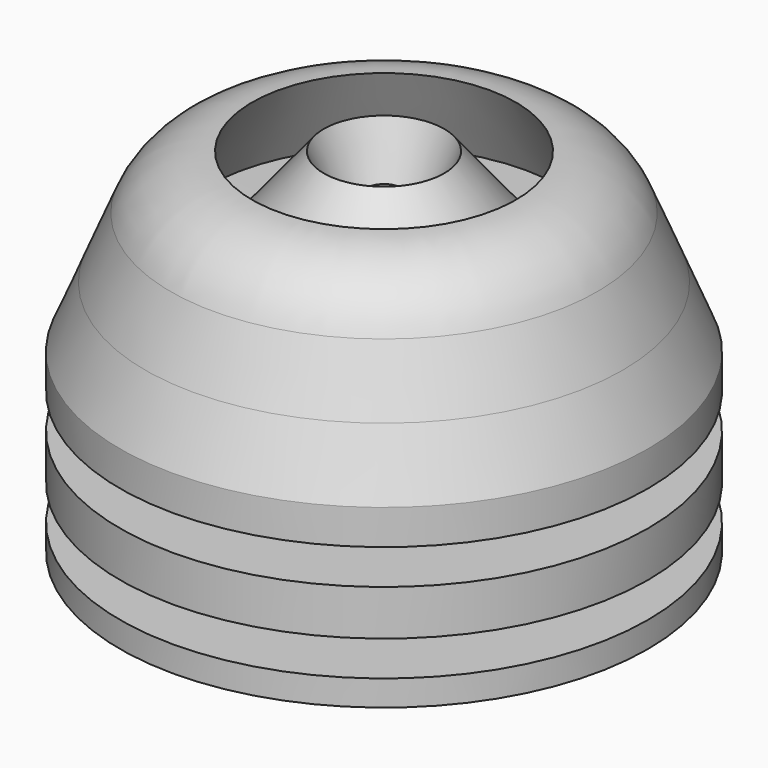
from build123d import *

# Parameters (mm, degrees)
F0_W   = 7.935712114
F0_H   = 3.1514726579
F0_W_2 = 16.216346994
F0_H_2 = 4.3113194406
F0_W_3 = 8.2806348801
F0_H_3 = 5.5851191282
F0_H_4 = 4.3113231659
F0_H_5 = 4.2968690395


with BuildPart() as f1:
    # F0 (on Right) → F1 (revolve)
    with BuildSketch(Plane.YZ):
        with Locations((20.184203051, 1.575736329)):
            Rectangle(F0_W, F0_H)
        with Locations((8.108173497, 5.3071323782)):
            Rectangle(F0_W_2, F0_H_2)
        with Locations((28.2923765481, 1.575736329)):
            Rectangle(F0_W_3, F0_H)
        with Locations((20.184203051, 5.3071323782)):
            Rectangle(F0_W, F0_H_2)
        with Locations((8.108173497, 10.2553516626)):
            Rectangle(F0_W_2, F0_H_3)
        with Locations((20.184203051, 10.2553516626)):
            Rectangle(F0_W, F0_H_3)
        with Locations((8.108173497, 15.2035728097)):
            Rectangle(F0_W_2, F0_H_4)
        with Locations((28.2923765481, 10.2553516626)):
            Rectangle(F0_W_3, F0_H_3)
        with Locations((20.184203051, 15.2035728097)):
            Rectangle(F0_W, F0_H_4)
        with Locations((8.108173497, 19.5076689124)):
            Rectangle(F0_W_2, F0_H_5)
        with Locations((20.184203051, 19.5076689124)):
            Rectangle(F0_W, F0_H_5)
        with BuildLine():
            Line((0, 39.0138179064), (0, 21.6561034322))
            Line((0, 21.6561034322), (16.216346994, 21.6561034322))
            Line((16.216346994, 21.6561034322), (16.216346994, 32.4841551483))
            Line((16.216346994, 32.4841551483), (7.3967017233, 43.3122068644))
            Line((7.3967017233, 43.3122068644), (3.9672423154, 34.0166091919))
            ThreePointArc((3.9672423154, 34.0166091919), (3.3885401848, 37.6305670459), (0, 39.0138179064))
        make_face()
        with Locations((28.2923765481, 19.5076689124)):
            Rectangle(F0_W_3, F0_H_5)
        with BuildLine():
            ThreePointArc((26.2175577062, 36.6341537335), (25.2214317596, 26.471239688), (16.216346994, 21.6561034322))
            Line((16.216346994, 21.6561034322), (24.152059108, 21.6561034322))
            Line((24.152059108, 21.6561034322), (32.4326939881, 21.6561034322))
            Line((32.4326939881, 21.6561034322), (29.3251258471, 29.1451285828))
            Line((29.3251258471, 29.1451285828), (26.2175577062, 36.6341537335))
        make_face()
        with BuildLine():
            Line((16.216346994, 32.4841551483), (16.216346994, 21.6561034322))
            ThreePointArc((16.216346994, 21.6561034322), (25.2214317596, 26.471239688), (26.2175577062, 36.6341537335))
            ThreePointArc((26.2175577062, 36.6341537335), (22.2292624543, 41.4892399138), (16.216346994, 43.3122068644))
            Line((16.216346994, 43.3122068644), (21.7024460435, 32.4488542974))
            Line((21.7024460435, 32.4488542974), (16.216346994, 32.4841551483))
        make_face()
    revolve(axis=Axis((0, 0, 21.6561034322), (0, 0, 1)))


solid = f1.part
